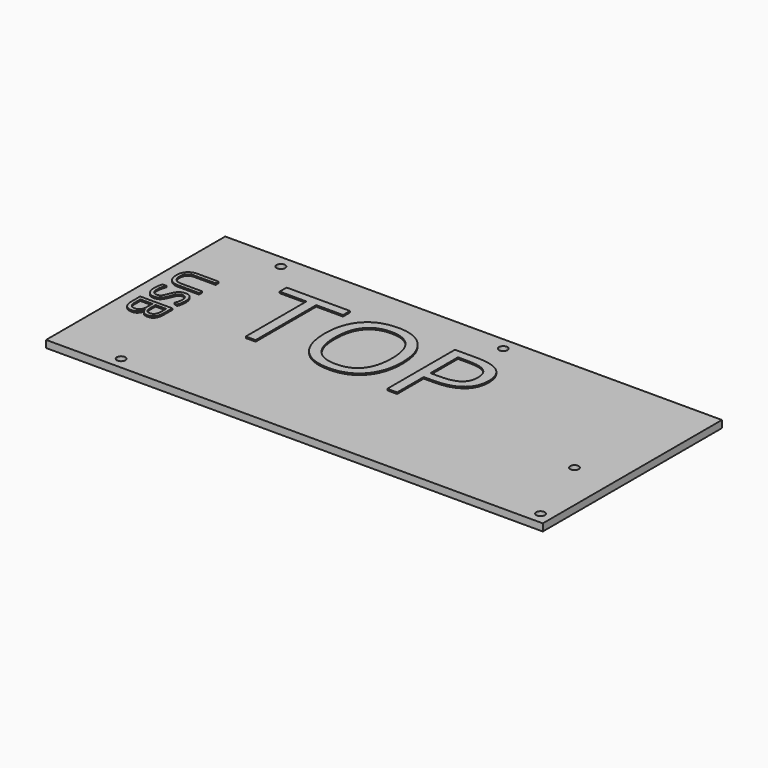
from build123d import *

# Parameters (mm, degrees)
F0_W           = 175.25
F0_H           = 79
F0_R           = 1.5
F1_DEPTH       = 2.54
F2_TEXT_SIZE   = 41.7767558247
F2_TEXT_SIZE_2 = 15.9005634487
F3_DEPTH       = 0.508


# Not quite as in the source:
# - Text() gives the source's letters only with a copy of the font that has no kerning and outlines rounded to 1/6400 em; it was checked with that copy


with BuildPart() as f1:
    # F0 (on Top) → F1 (new body)
    with BuildSketch(Plane.XY):
        with Locations((87.625, 39.5)):
            Rectangle(F0_W, F0_H)
        with Locations((23.18, 4.11)):
            Circle(F0_R, mode=Mode.SUBTRACT)
        with Locations((171.18, 4.11)):
            Circle(F0_R, mode=Mode.SUBTRACT)
        with Locations((161.29, 31.43)):
            Circle(F0_R, mode=Mode.SUBTRACT)
        with Locations((23.18, 74.6)):
            Circle(F0_R, mode=Mode.SUBTRACT)
        with Locations((101.6, 74.6)):
            Circle(F0_R, mode=Mode.SUBTRACT)
    extrude(amount=F1_DEPTH)

    # F2 (on face) → F3 (join)
    with BuildSketch(Plane.XY.offset(2.54)):
        with Locations((32.4909426272, 35.1921282709)):
            Text('TOP', F2_TEXT_SIZE, font='Open Sans', text_align=(TextAlign.LEFT, TextAlign.BOTTOM))
        with Locations(Location((4.6582822688, 57.5326345861), (0, 0, -90))):
            Text('USB', F2_TEXT_SIZE_2, font='Open Sans', text_align=(TextAlign.LEFT, TextAlign.BOTTOM))
    extrude(amount=F3_DEPTH)


solid = f1.part
